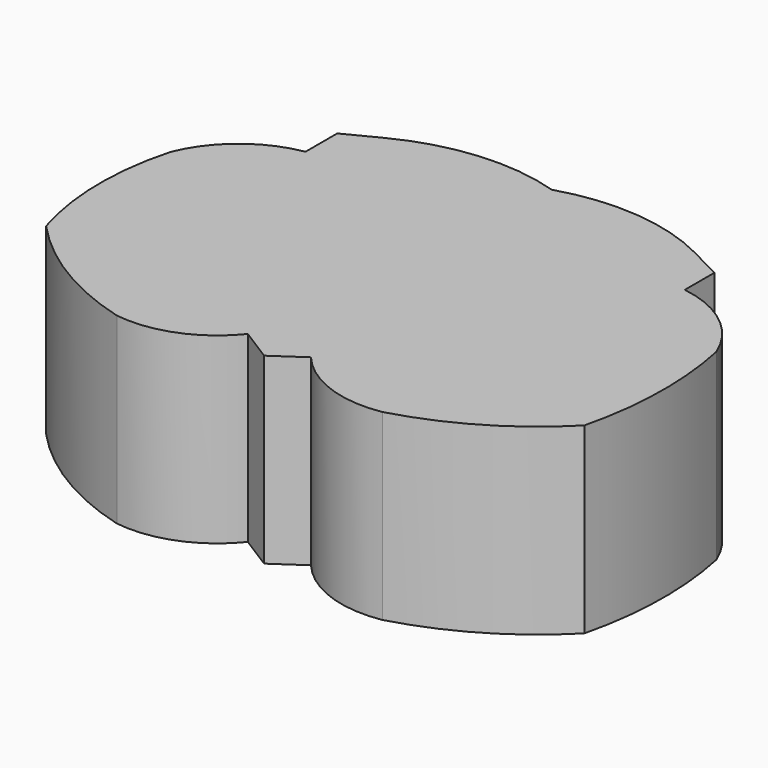
from build123d import *

# Parameters (mm, degrees)
F1_DEPTH = 11.90625


# Not quite as in the source:
# - a length typed as a fraction of an inch, garbled in the dataset ("3 / 203.2 mm" for 3/8 in), is restored


with BuildPart() as f1:
    # F0 (on Top) → F1 (new body)
    with BuildSketch(Plane.XY):
        with BuildLine():
            ThreePointArc((0, 9.1178910807), (-5.1898410508, 9.6890057882), (-10.2093555033, 8.2519613206))
            Line((-10.2093555033, 8.2519613206), (-12.369341217, 7.1464567445))
            Line((-12.369341217, 7.1464567445), (-12.369341217, 4.6386048198))
            Line((-12.369341217, 4.6386048198), (-12.369341217, 4.5682978211))
            ThreePointArc((-12.369341217, 4.5682978211), (-15.5930977879, 3.1185654947), (-17.7027139134, 0.2823972963))
            ThreePointArc((-17.7027139134, 0.2823972963), (-18.3641606661, -4.889059653), (-17.5542831421, -10.0393583998))
            ThreePointArc((-17.5542831421, -10.0393583998), (-13.4613837791, -13.3941238354), (-8.5996589687, -15.484556372))
            ThreePointArc((-8.5996589687, -15.484556372), (-5.0294162563, -15.0523544446), (-2.1409380715, -12.9098966718))
            Line((-2.1409380715, -12.9098966718), (0, -14.2561570176))
            Line((0, -14.2561570176), (1.9696742658, -12.9098966718))
            ThreePointArc((1.9696742658, -12.9098966718), (4.9392756736, -15.0084468105), (8.560301624, -15.3410370587))
            ThreePointArc((8.560301624, -15.3410370587), (13.367982191, -13.3015402533), (17.4874793738, -10.0916987285))
            ThreePointArc((17.4874793738, -10.0916987285), (18.16772005, -4.8427956267), (17.6633565687, 0.4259166096))
            ThreePointArc((17.6633565687, 0.4259166096), (15.4847616458, 3.3168082822), (12.1560195839, 4.739132713))
            Line((12.1560195839, 4.739132713), (12.1560195839, 7.1464567445))
            Line((12.1560195839, 7.1464567445), (9.9960338703, 8.2519613206))
            ThreePointArc((9.9960338703, 8.2519613206), (5.0827762692, 9.6633625741), (0, 9.1178910807))
        make_face()
    extrude(amount=F1_DEPTH)


solid = f1.part
